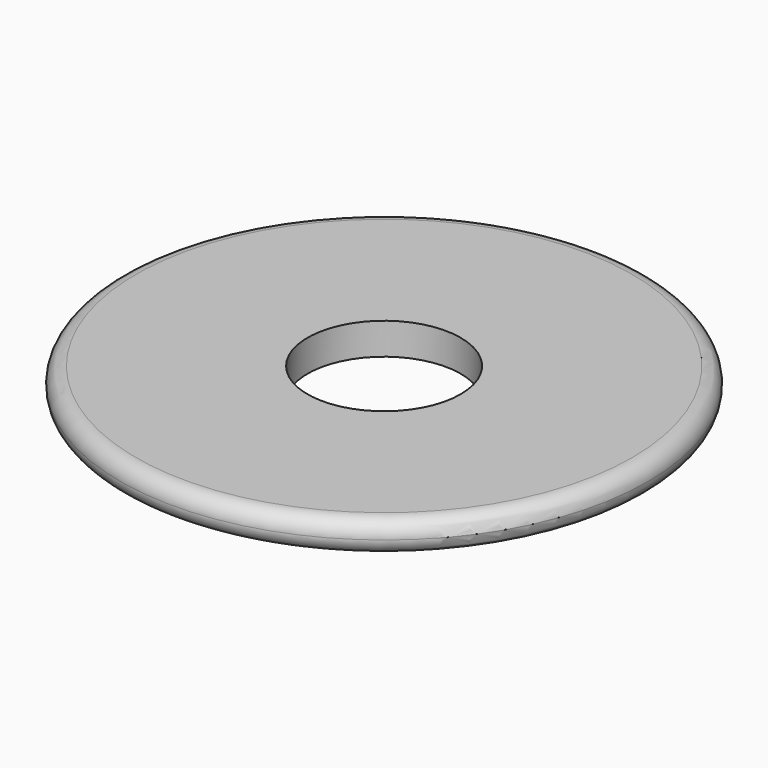
from build123d import *

# Parameters (mm, degrees)
F0_R     = 12.7
F0_R_2   = 3.683
F1_DEPTH = 1.524
F2_R     = 0.76199


# Not quite as in the source:
# - a fillet or chamfer is up to 0.001 mm smaller than in the source, because OpenCascade refuses the exact size


with BuildPart() as f1:
    # F0 (on Top) → F1 (new body)
    with BuildSketch(Plane.XY):
        Circle(F0_R)
        Circle(F0_R_2, mode=Mode.SUBTRACT)
    extrude(amount=F1_DEPTH)

    # F2 (radius 0.762 in the source; OpenCascade refuses exactly that, so slightly less here)
    f2_edges = [f1.edges().sort_by_distance(p)[0] for p in [
        (-12.7, 0, 1.524),
        (-12.7, 0, 0),
    ]]
    fillet(f2_edges, radius=F2_R)


solid = f1.part
